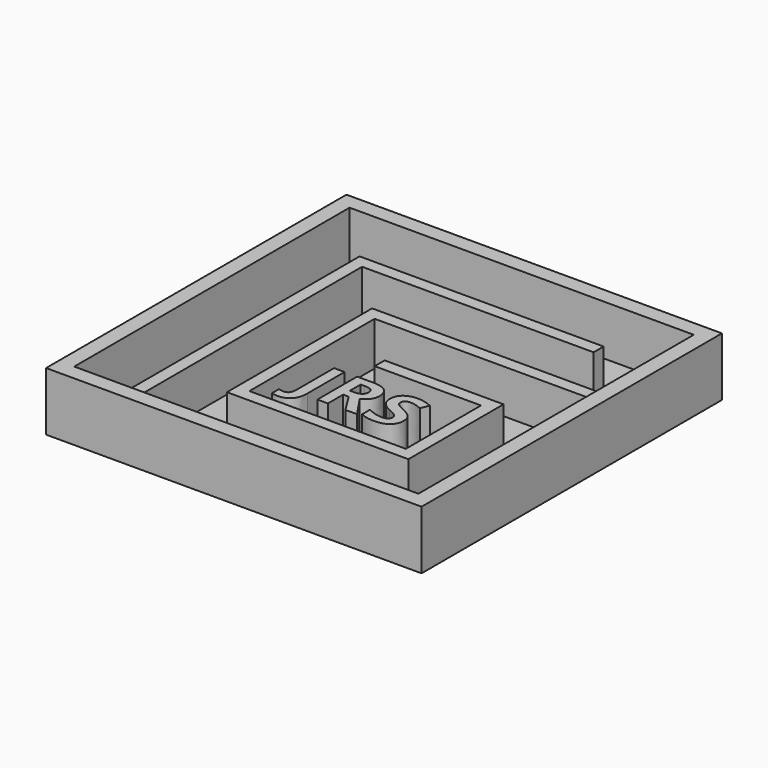
from build123d import *

# Parameters (mm, degrees)
F0_W         = 38.1
F0_H         = 38.1
F1_DEPTH     = 0.079375
F2_W         = 38.1
F2_H         = 38.1
F2_W_2       = 34.925
F2_H_2       = 34.925
F3_DEPTH     = 5.08
F4_W         = 23.495
F4_H         = 1.27
F4_W_2       = 10.795
F5_DEPTH     = 4.445
F6_DEPTH     = 0.79375
F7_TEXT_SIZE = 7.0555555556
F8_DEPTH     = 4.445
F4_R         = 1.27
F9_DEPTH     = 0.396875


# Not quite as in the source:
# - a feature names something its author has since deleted; it is built from what else it names
# - Text() gives the source's letters only with a copy of the font that has no kerning and outlines rounded to 1/6400 em; it was checked with that copy


with BuildPart() as f1:
    # F0 (on Top) → F1 (new body)
    with BuildSketch(Plane.XY):
        with Locations((-1.7210580409, -0.9158205878)):
            Rectangle(F0_W, F0_H)
    extrude(amount=F1_DEPTH)

    # F2 (on face) → F3 (join)
    with BuildSketch(Plane.XY.offset(0.079375)):
        with Locations((-1.7210580409, -0.9158205878)):
            Rectangle(F2_W, F2_H)
        with Locations((-1.7210580409, -0.9158205878)):
            Rectangle(F2_W_2, F2_H_2, mode=Mode.SUBTRACT)
    extrude(amount=F3_DEPTH)

    # F4 (on face) → F5 (join)
    with BuildSketch(Plane.XY.offset(0.079375)):
        with Locations((-1.0860580409, 10.8316794122)):
            Rectangle(F4_W, F4_H)
        Polygon((-6.4835580409, 3.8466794122), (15.7414419591, 3.8466794122), (15.7414419591, 5.1166794122), (-7.7535580409, 5.1166794122), (-7.7535580409, 3.8466794122), align=None)
        Polygon((-6.4835580409, -12.0358048007), (-6.4835580409, 3.8466794122), (-7.7535580409, 3.8466794122), (-7.7535580409, -13.2983205878), (-6.4835580409, -13.2983205878), align=None)
        Polygon((-14.1035580409, 11.4666794122), (-14.1035580409, -18.3783205878), (-12.8335580409, -18.3783205878), (-12.8335580409, 10.1966794122), (-12.8335580409, 11.4666794122), align=None)
        with Locations((3.9939419591, -1.8683205878)):
            Rectangle(F4_W_2, F4_H)
        Polygon((9.3914419591, -2.5033205878), (9.3914419591, -12.0358048007), (10.6614419591, -12.0358048007), (10.6614419591, -1.2333205878), (9.3914419591, -1.2333205878), align=None)
        Polygon((9.3914419591, -12.0358048007), (-6.4835580409, -12.0358048007), (-6.4835580409, -13.2983205878), (10.6614419591, -13.2983205878), (10.6614419591, -12.0358048007), align=None)
    extrude(amount=F5_DEPTH)

    # F0 (on Top) → F6 (join)
    with BuildSketch(Plane.XY):
        with Locations((-1.7210580409, -0.9158205878)):
            Rectangle(F0_W, F0_H)
    extrude(amount=-F6_DEPTH)

    # F7 (on face) → F8 (join)
    with BuildSketch(Plane.XY.offset(0.079375)):
        with Locations((-4.3371257492, -9.8095626942)):
            Text('JRS', F7_TEXT_SIZE, font='Open Sans', font_style=FontStyle.BOLD, text_align=(TextAlign.LEFT, TextAlign.BOTTOM))
    extrude(amount=F8_DEPTH)

    # F4 (on face) → F9 (cut)
    with BuildSketch(Plane.XY.offset(0.079375)):
        with Locations((-16.6435580409, -15.8383205878)):
            Circle(F4_R)
        with Locations((-3.9435580409, -1.2333205878)):
            Circle(F4_R)
    extrude(amount=-F9_DEPTH, mode=Mode.SUBTRACT)


solid = f1.part
